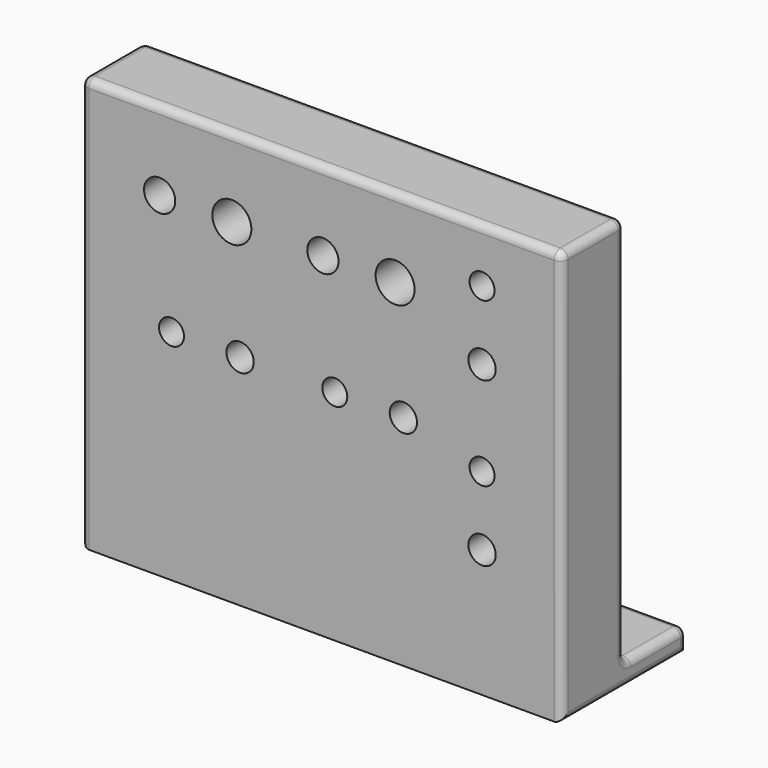
from build123d import *

# Parameters (mm, degrees)
F0_W          = 100
F0_H          = 5
F1_DEPTH      = 3
F2_W          = 100
F2_H          = 10
F3_DEPTH      = 50
F4_R          = 1.6
F4_R_2        = 1.75
F4_R_3        = 2.5
F4_R_4        = 2
F5_DEPTH      = 50
F7_DEPTH      = 50
F7_DEPTH_BACK = 25
F8_R          = 1


with BuildPart() as f1:
    # F0 (on Top) → F1 (new body)
    with BuildSketch(Plane.XY):
        with Locations((0, 12.6435890049)):
            Rectangle(F0_W, F0_H)
        with Locations((0, 7.6435890049)):
            Rectangle(F0_W, F0_H)
        with Locations((0, 2.6435890049)):
            Rectangle(F0_W, F0_H)
        with Locations((0, -2.3564109951)):
            Rectangle(F0_W, F0_H)
    extrude(amount=F1_DEPTH)

    # F2 (on face) → F3 (join)
    with BuildSketch(Plane.XY.offset(3)):
        with Locations((0, 0.1435890049)):
            Rectangle(F2_W, F2_H)
    extrude(amount=F3_DEPTH)

    # F4 (on face) → F5 (cut)
    with BuildSketch(Plane.XZ.offset(4.8564109951)):
        with Locations((0, 28)):
            Circle(F4_R)
        with Locations((39.7706801567, 25.1996132218)):
            Circle(F4_R)
        with Locations((8.7829349406, 28)):
            Circle(F4_R_2)
        with Locations((39.7706801567, 37.2641024557)):
            Circle(F4_R_2)
        with Locations((20.9091, 28)):
            Circle(F4_R)
        with Locations((29.6920349406, 28)):
            Circle(F4_R_2)
        with Locations((39.7706801567, 46.1087132218)):
            Circle(F4_R)
        with Locations((39.7706801567, 16.3550024557)):
            Circle(F4_R_2)
        with Locations((7.7257619488, 42.9009612363)):
            Circle(F4_R_3)
        with Locations((28.6348619488, 42.9009612363)):
            Circle(F4_R_3)
        with Locations((-1.5212555765, 42.9009612363)):
            Circle(F4_R_4)
        with Locations((19.3878444235, 42.9009612363)):
            Circle(F4_R_4)
    extrude(amount=-F5_DEPTH, mode=Mode.SUBTRACT)

    # F6 (on face) → F7 (cut, two sides)
    with BuildSketch(Plane.XZ.offset(4.8564109951)) as f7_sk:
        Polygon((-50, 53), (-11.575919576, 53), (-11.575919576, 62.5623986125), (-61.6087988019, 62.5623986125), (-61.6087988019, -15.408792533), (-11.575919576, -17.8658775985), (-11.575919576, 0), (-50, 0), align=None)
        Polygon((-11.575919576, 0), (-11.575919576, 49.896787852), (-11.575919576, 53), (-50, 53), (-50, 0), align=None)
    extrude(amount=-F7_DEPTH, mode=Mode.SUBTRACT)
    extrude(f7_sk.sketch, amount=F7_DEPTH_BACK, mode=Mode.SUBTRACT)

    # F8
    f8_edges = [f1.edges().sort_by_distance(p)[0] for p in [
        (50, -4.856411, 26.5),
        (50, 0.143589, 53),
        (50, 5.143589, 28),
        (50, 10.143589, 3),
        (50, 15.143589, 1.5),
        (50, 5.143589, 0),
        (-11.57592, 0.143589, 53),
        (19.21204, 5.143589, 53),
        (19.21204, -4.856411, 53),
        (-11.57592, 5.143589, 0),
        (-11.57592, -4.856411, 26.5),
        (-11.57592, 5.143589, 28),
        (-11.57592, 10.143589, 3),
        (-11.57592, 15.143589, 1.5),
        (19.21204, 5.143589, 3),
        (19.21204, 15.143589, 3),
    ]]
    fillet(f8_edges, radius=F8_R)


solid = f1.part
